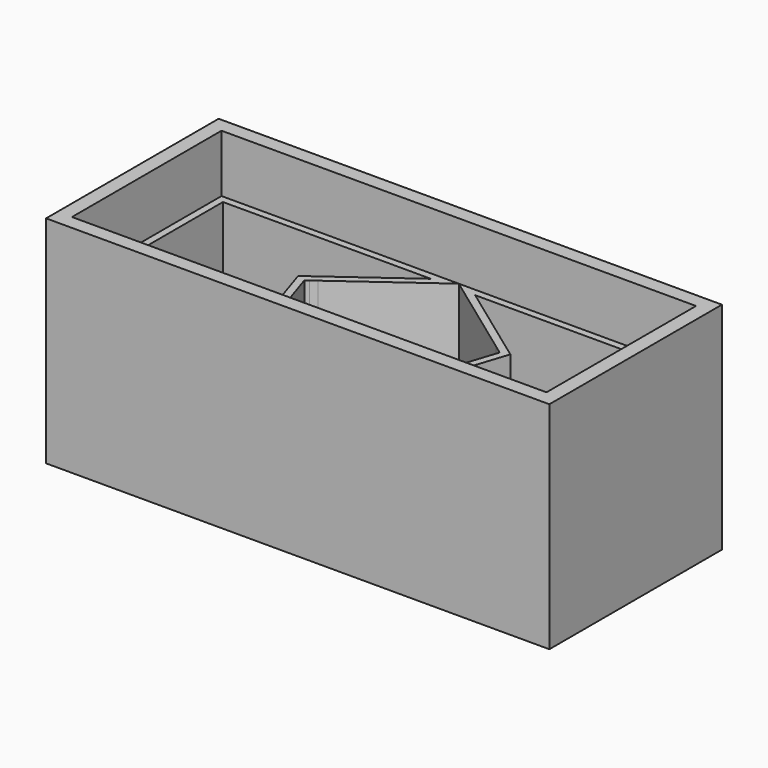
from build123d import *

# Parameters (mm, degrees)
F0_W     = 88.9
F0_H     = 38.1
F1_DEPTH = 38.1
F2_T     = -2.54
F4_DEPTH = 25.4
F5_T     = -1.27
F6_T     = -1.27


with BuildPart() as f1:
    # F0 (on Top) → F1 (new body)
    with BuildSketch(Plane.XY):
        Rectangle(F0_W, F0_H)
    extrude(amount=F1_DEPTH)

    # F2
    f2_openings = [f1.faces().sort_by_distance(p)[0] for p in [
        (0, 0, 38.1),
    ]]
    offset(amount=F2_T, openings=f2_openings)


with BuildPart() as f4:
    # F3 (on face) → F4 (new body)
    with BuildSketch(Plane.XY.offset(2.54)):
        Polygon((-15.701943084, 5.1018705771), (0, 16.51), (-41.91, 16.51), (-41.91, -16.51), (-10.5966423781, -16.51), (-17.2526844283, 3.9751910406), (-16.6781271043, 4.3926313713), align=None)
    extrude(amount=F4_DEPTH)

    # F5
    f5_openings = [f4.faces().sort_by_distance(p)[0] for p in [
        (-26.606347, 0.679846, 27.94),
    ]]
    offset(amount=F5_T, openings=f5_openings, kind=Kind.INTERSECTION)


with BuildPart() as f4b:
    # F3 (on face) → F4, piece 2 (new body)
    with BuildSketch(Plane.XY.offset(2.54)):
        Polygon((41.91, 16.51), (0, 16.51), (15.701943084, 5.1018705771), (16.6781271043, 4.3926313713), (17.2526844283, 3.9751910406), (10.5966423781, -16.51), (41.91, -16.51), align=None)
    extrude(amount=F4_DEPTH)

    # F6
    f6_openings = [f4b.faces().sort_by_distance(p)[0] for p in [
        (26.606347, 0.679846, 27.94),
    ]]
    offset(amount=F6_T, openings=f6_openings, kind=Kind.INTERSECTION)


solid = Compound([f1.part, f4.part, f4b.part])
